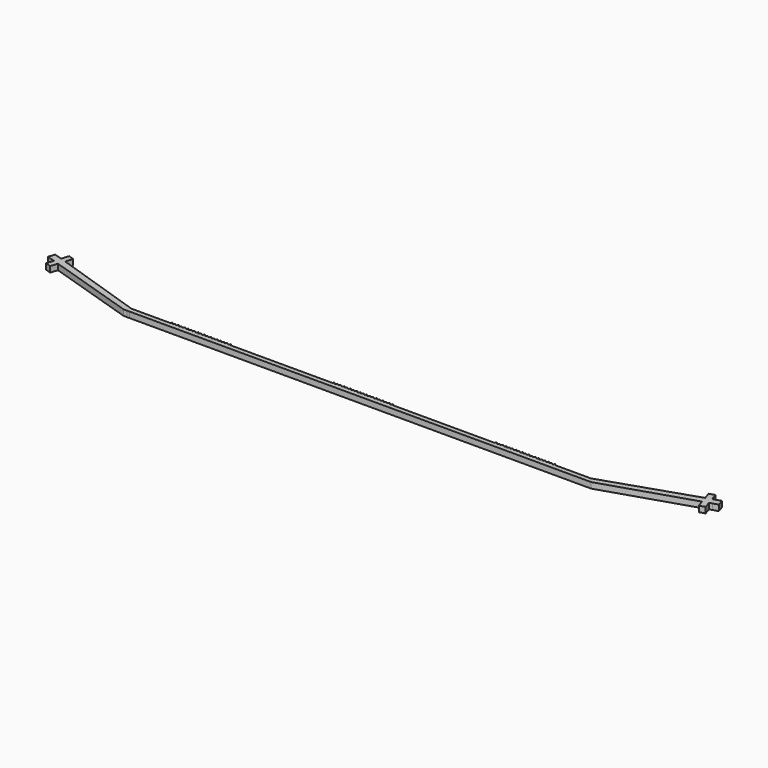
from build123d import *

# Parameters (mm, degrees)
F1_DEPTH = 4.45


# Not quite as in the source:
# - ends of sketch curves that miss each other by under 0.0002 mm in the source are joined


with BuildPart() as f1:
    # F0 (on Top) → F1 (new body)
    with BuildSketch(Plane.XY):
        Polygon((-262.717832135, 10.3832809954), (-260.7070284328, 10.3832819745), (94.8929715672, 10.3832819745), (162.8652340118, 32.1849133881), (164.5834296942, 26.8279910088), (168.8208022167, 28.187098843), (167.1026050773, 33.544025765), (169.2707606129, 34.2394466086), (173.1350229335, 35.4788819345), (171.5514059448, 40.416220198), (165.5048181879, 38.4768191312), (163.7239287988, 44.0292054635), (159.4865562763, 42.6700976293), (161.2674456653, 37.117711297), (91.7756564294, 14.0403658152), (64.2810454752, 14.0403658152), (63.4150589707, 15.1818566933), (62.5490724606, 14.0403658152), (61.7810454752, 14.0403658152), (60.9150589707, 15.1818566933), (60.0490724606, 14.0403658152), (59.2810454752, 14.0403658152), (58.4150589707, 15.1818566933), (57.5490724606, 14.0403658152), (56.7810454752, 14.0403658152), (55.9150589707, 15.1818566933), (55.0490724606, 14.0403658152), (54.2810454752, 14.0403658152), (53.4150589707, 15.1818566933), (52.5490724606, 14.0403658152), (51.7810454752, 14.0403658152), (50.9150589707, 15.1818566933), (50.0490724606, 14.0403658152), (49.2810454752, 14.0403658152), (48.4150589707, 15.1818566933), (47.5490724606, 14.0403658152), (46.7810454752, 14.0403658152), (45.9150589707, 15.1818566933), (45.0490724606, 14.0403658152), (44.2810454752, 14.0403658152), (43.4150589707, 15.1818566933), (42.5490724606, 14.0403658152), (41.7810454752, 14.0403658152), (40.9150589707, 15.1818566933), (40.0490724606, 14.0403658152), (39.2810454752, 14.0403658152), (38.4150589707, 15.1818566933), (37.5490724606, 14.0403658152), (36.7810454752, 14.0403658152), (35.9150589707, 15.1818566933), (35.0490724606, 14.0403658152), (34.2810454752, 14.0403658152), (33.4150589707, 15.1818566933), (32.5490724606, 14.0403658152), (31.7810454752, 14.0403658152), (30.9150589707, 15.1818566933), (30.0490724606, 14.0403658152), (29.2810454752, 14.0403658152), (28.4150589707, 15.1818566933), (27.5490724606, 14.0403658152), (26.7810454752, 14.0403658152), (25.9150589707, 15.1818566933), (25.0490724606, 14.0403658152), (24.2810454752, 14.0403658152), (23.4150589707, 15.1818566933), (22.5490724606, 14.0403658152), (21.7810454752, 14.0403658152), (20.9150589707, 15.1818566933), (20.0490724606, 14.0403658152), (19.2810454752, 14.0403658152), (18.4150589707, 15.1818566933), (17.5490724606, 14.0403658152), (-60.7189545248, 14.0403658152), (-61.5849410293, 15.1818566933), (-62.4509275394, 14.0403658152), (-63.2189545248, 14.0403658152), (-64.0849410293, 15.1818566933), (-64.9509275394, 14.0403658152), (-65.7189545248, 14.0403658152), (-66.5849410293, 15.1818566933), (-67.4509275394, 14.0403658152), (-68.2189545248, 14.0403658152), (-69.0849410293, 15.1818566933), (-69.9509275394, 14.0403658152), (-70.7189545248, 14.0403658152), (-71.5849410293, 15.1818566933), (-72.4509275394, 14.0403658152), (-73.2189545248, 14.0403658152), (-74.0849410293, 15.1818566933), (-74.9509275394, 14.0403658152), (-75.7189545248, 14.0403658152), (-76.5849410293, 15.1818566933), (-77.4509275394, 14.0403658152), (-78.2189545248, 14.0403658152), (-79.0849410293, 15.1818566933), (-79.9509275394, 14.0403658152), (-80.7189545248, 14.0403658152), (-81.5849410293, 15.1818566933), (-82.4509275394, 14.0403658152), (-83.2189545248, 14.0403658152), (-84.0849410293, 15.1818566933), (-84.9509275394, 14.0403658152), (-85.7189545248, 14.0403658152), (-86.5849410293, 15.1818566933), (-87.4509275394, 14.0403658152), (-88.2189545248, 14.0403658152), (-89.0849410293, 15.1818566933), (-89.9509275394, 14.0403658152), (-90.7189545248, 14.0403658152), (-91.5849410293, 15.1818566933), (-92.4509275394, 14.0403658152), (-93.2189545248, 14.0403658152), (-94.0849410293, 15.1818566933), (-94.9509275394, 14.0403658152), (-95.7189545248, 14.0403658152), (-96.5849410293, 15.1818566933), (-97.4509275394, 14.0403658152), (-98.2189545248, 14.0403658152), (-99.0849410293, 15.1818566933), (-99.9509275394, 14.0403658152), (-100.7189545248, 14.0403658152), (-101.5849410293, 15.1818566933), (-102.4509275394, 14.0403658152), (-103.2189545248, 14.0403658152), (-104.0849410293, 15.1818566933), (-104.9509275394, 14.0403658152), (-105.7189545248, 14.0403658152), (-106.5849410293, 15.1818566933), (-107.4509275394, 14.0403658152), (-185.7189545248, 14.0403658152), (-186.5849410293, 15.1818566933), (-187.4509275394, 14.0403658152), (-188.2189545248, 14.0403658152), (-189.0849410293, 15.1818566933), (-189.9509275394, 14.0403658152), (-190.7189545248, 14.0403658152), (-191.5849410293, 15.1818566933), (-192.4509275394, 14.0403658152), (-193.2189545248, 14.0403658152), (-194.0849410293, 15.1818566933), (-194.9509275394, 14.0403658152), (-195.7189545248, 14.0403658152), (-196.5849410293, 15.1818566933), (-197.4509275394, 14.0403658152), (-198.2189545248, 14.0403658152), (-199.0849410293, 15.1818566933), (-199.9509275394, 14.0403658152), (-200.7189545248, 14.0403658152), (-201.5849410293, 15.1818566933), (-202.4509275394, 14.0403658152), (-203.2189545248, 14.0403658152), (-204.0849410293, 15.1818566933), (-204.9509275394, 14.0403658152), (-205.7189545248, 14.0403658152), (-206.5849410293, 15.1818566933), (-207.4509275394, 14.0403658152), (-208.2189545248, 14.0403658152), (-209.0849410293, 15.1818566933), (-209.9509275394, 14.0403658152), (-210.7189545248, 14.0403658152), (-211.5849410293, 15.1818566933), (-212.4509275394, 14.0403658152), (-213.2189545248, 14.0403658152), (-214.0849410293, 15.1818566933), (-214.9509275394, 14.0403658152), (-215.7189545248, 14.0403658152), (-216.5849410293, 15.1818566933), (-217.4509275394, 14.0403658152), (-218.2189545248, 14.0403658152), (-219.0849410293, 15.1818566933), (-219.9509275394, 14.0403658152), (-220.7189545248, 14.0403658152), (-221.5849410293, 15.1818566933), (-222.4509275394, 14.0403658152), (-223.2189545248, 14.0403658152), (-224.0849410293, 15.1818566933), (-224.9509275394, 14.0403658152), (-225.7189545248, 14.0403658152), (-226.5849410293, 15.1818566933), (-227.4509275394, 14.0403658152), (-228.2189545248, 14.0403658152), (-229.0849410293, 15.1818566933), (-229.9509275394, 14.0403658152), (-230.7189545248, 14.0403658152), (-231.5849410293, 15.1818566933), (-232.4509275394, 14.0403658152), (-259.945538523, 14.0403658152), (-262.1965405745, 14.0403653266), (-331.6883298105, 37.1177104356), (-329.9074404214, 42.6700967679), (-334.144812944, 44.0292046021), (-335.9257023331, 38.4768182698), (-341.97229009, 40.4162193366), (-343.5559070786, 35.4788810731), (-339.6916447581, 34.2394457472), (-337.5234892224, 33.5440249036), (-339.2416863619, 28.1870979816), (-335.0043138393, 26.8279901474), (-333.2861181569, 32.1849125267), (-265.3138557124, 10.3832809954), align=None)
    extrude(amount=F1_DEPTH)


solid = f1.part
